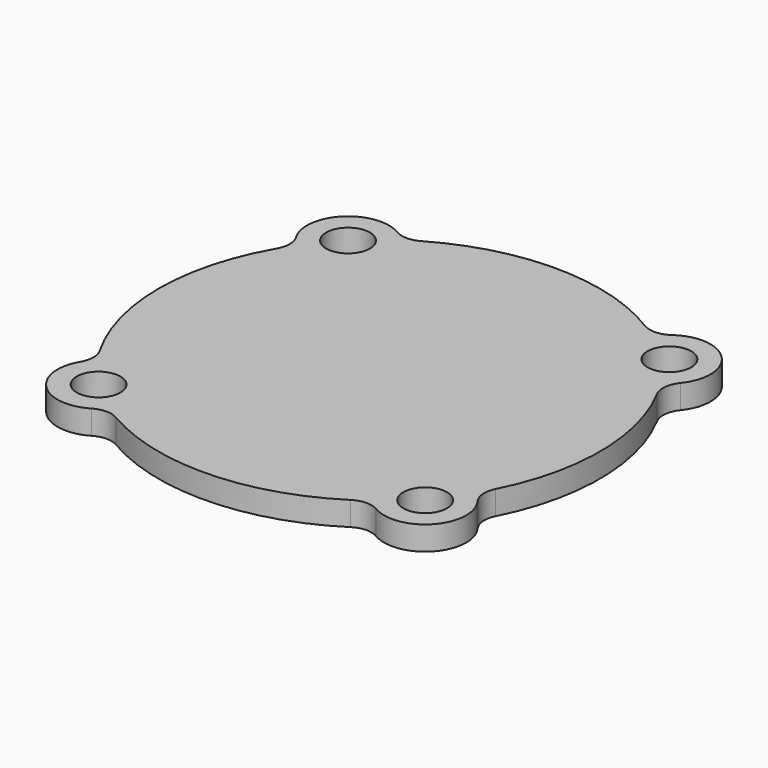
from build123d import *

# Parameters (mm, degrees)
F0_R     = 5.7785
F1_DEPTH = 6.35
F2_R     = 6.35


with BuildPart() as f1:
    # F0 (on Top) → F1 (new body)
    with BuildSketch(Plane.XY):
        with BuildLine():
            ThreePointArc((-32.9470856511, 48.2429885797), (-48.9531189835, 48.9531189835), (-48.2429885797, 32.9470856511))
            ThreePointArc((-48.2429885797, 32.9470856511), (-58.42, 0), (-48.2429885797, -32.9470856511))
            ThreePointArc((-48.2429885797, -32.9470856511), (-48.9531189835, -48.9531189835), (-32.9470856511, -48.2429885797))
            ThreePointArc((-32.9470856511, -48.2429885797), (1.5282374195, -58.4000076232), (35.4251532331, -46.4537933695))
            ThreePointArc((35.4251532331, -46.4537933695), (51.8744333617, -46.8373507019), (49.8184745785, -30.5125546401))
            ThreePointArc((49.8184745785, -30.5125546401), (58.4153919217, 0.7337483426), (49.0363490334, 31.7542575646))
            ThreePointArc((49.0363490334, 31.7542575646), (51.7187959431, 48.720604874), (34.622654511, 47.0549486729))
            ThreePointArc((34.622654511, 47.0549486729), (1.0270065512, 58.4109720647), (-32.9470856511, 48.2429885797))
        make_face()
        with Locations((-41.275, -41.275)):
            Circle(F0_R, mode=Mode.SUBTRACT)
        with Locations((43.815, -39.5605)):
            Circle(F0_R, mode=Mode.SUBTRACT)
        with Locations((-41.275, 41.275)):
            Circle(F0_R, mode=Mode.SUBTRACT)
        with Locations((43.815, 41.275)):
            Circle(F0_R, mode=Mode.SUBTRACT)
    extrude(amount=F1_DEPTH)

    # F2
    f2_edges = [f1.edges().sort_by_distance(p)[0] for p in [
        (-48.242989, 32.947086, 3.175),
        (35.425153, -46.453793, 3.175),
        (49.818475, -30.512555, 3.175),
        (-32.947086, 48.242989, 3.175),
        (34.622655, 47.054949, 3.175),
        (49.036349, 31.754258, 3.175),
        (-48.242989, -32.947086, 3.175),
        (-32.947086, -48.242989, 3.175),
    ]]
    fillet(f2_edges, radius=F2_R)


solid = f1.part
